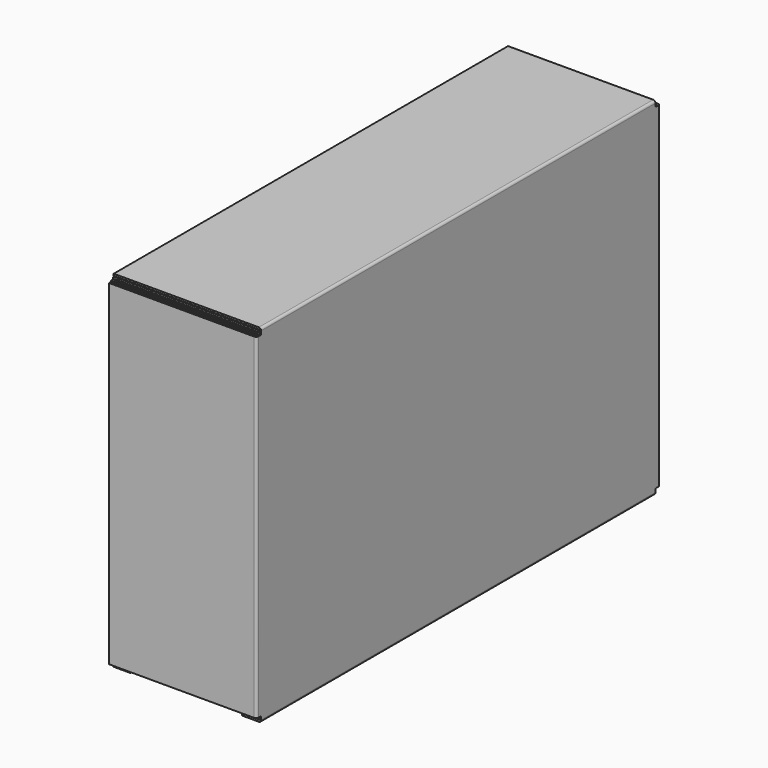
from build123d import *

# Parameters (mm, degrees)
F0_W      = 1092.2
F0_H      = 749.3
F1_DEPTH  = 317.5
F2_T      = -4.064
F3_W      = 279.4
F3_H      = 1717.7925925926
F4_DEPTH  = 4.064
F6_DEPTH  = 317.501
F7_R      = 2.54
F8_W      = 1084.072
F8_H      = 12.7
F9_DEPTH  = 313.436
F10_DEPTH = 317.5
F11_T     = 4.064
F13_DEPTH = 321.565
F14_R     = 5.08
F15_W     = 279.4
F15_H     = 1074.928
F16_DEPTH = 25.4


with BuildPart() as f1:
    # F0 (on Right) → F1 (new body)
    with BuildSketch(Plane.YZ):
        with Locations((546.1, 374.65)):
            Rectangle(F0_W, F0_H)
    extrude(amount=F1_DEPTH)

    # F2
    f2_openings = [f1.faces().sort_by_distance(p)[0] for p in [
        (317.5, 546.1, 374.65),
    ]]
    offset(amount=F2_T, openings=f2_openings)

    # F3 (on face) → F4 (cut)
    with BuildSketch(Plane(origin=(0, 0, 0), x_dir=(1, 0, 0), z_dir=(0, 0, -1))):
        with Locations((177.8, -858.8962962963)):
            Rectangle(F3_W, F3_H)
    extrude(amount=-F4_DEPTH, mode=Mode.SUBTRACT)

    # F5 (on face) → F6 (cut, through all)
    with BuildSketch(Plane(origin=(0, 0, 0), x_dir=(0, -1, 0), z_dir=(-1, 0, 0))):
        with BuildLine():
            Line((-1092.2, 6.35), (-1092.2, 0))
            Line((-1092.2, 0), (-1085.85, 0))
            Line((-1085.85, 0), (-1085.85, 3.81))
            ThreePointArc((-1085.85, 3.81), (-1086.5939487758, 5.6060512242), (-1088.39, 6.35))
            Line((-1088.39, 6.35), (-1092.2, 6.35))
        make_face()
        with BuildLine():
            Line((-1085.85, 749.3), (-1092.2, 749.3))
            Line((-1092.2, 749.3), (-1092.2, 742.95))
            Line((-1092.2, 742.95), (-1088.39, 742.95))
            ThreePointArc((-1088.39, 742.95), (-1086.5939487758, 743.6939487758), (-1085.85, 745.49))
            Line((-1085.85, 745.49), (-1085.85, 749.3))
        make_face()
        with BuildLine():
            Line((0, 742.95), (0, 749.3))
            Line((0, 749.3), (-6.35, 749.3))
            Line((-6.35, 749.3), (-6.35, 745.49))
            ThreePointArc((-6.35, 745.49), (-5.6060512242, 743.6939487758), (-3.81, 742.95))
            Line((-3.81, 742.95), (0, 742.95))
        make_face()
        with BuildLine():
            Line((-6.35, 0), (0, 0))
            Line((0, 0), (0, 6.35))
            Line((0, 6.35), (-3.81, 6.35))
            ThreePointArc((-3.81, 6.35), (-5.6060512242, 5.6060512242), (-6.35, 3.81))
            Line((-6.35, 3.81), (-6.35, 0))
        make_face()
    extrude(amount=-F6_DEPTH, mode=Mode.SUBTRACT)

    # F7
    f7_edges = [f1.edges().sort_by_distance(p)[0] for p in [
        (0, 1092.2, 374.65),
        (0, 546.1, 0),
        (0, 0, 374.65),
        (0, 546.1, 749.3),
    ]]
    fillet(f7_edges, radius=F7_R)


with BuildPart() as f9:
    # F8 (on face) → F9 (new body, through all)
    with BuildSketch(Plane.YZ.offset(4.064)):
        with Locations((546.1, 10.414)):
            Rectangle(F8_W, F8_H)
    extrude(amount=F9_DEPTH)


with BuildPart() as f10:
    # F0 (on Right) → F10 (new body)
    with BuildSketch(Plane.YZ):
        with Locations((546.1, 374.65)):
            Rectangle(F0_W, F0_H)
    extrude(amount=F10_DEPTH)

    # F11
    f11_openings = [f10.faces().sort_by_distance(p)[0] for p in [
        (0, 546.1, 374.65),
    ]]
    offset(amount=F11_T, openings=f11_openings, kind=Kind.INTERSECTION)

    # F12 (on face) → F13 (cut, through all)
    with BuildSketch(Plane.YZ.offset(321.564)):
        with BuildLine():
            Line((1083.564, -4.064), (1096.264, -4.064))
            Line((1096.264, -4.064), (1096.264, 8.636))
            Line((1096.264, 8.636), (1086.104, 8.636))
            ThreePointArc((1086.104, 8.636), (1084.3079487758, 7.8920512242), (1083.564, 6.096))
            Line((1083.564, 6.096), (1083.564, -4.064))
        make_face()
        with BuildLine():
            Line((8.636, 753.364), (-4.064, 753.364))
            Line((-4.064, 753.364), (-4.064, 740.664))
            Line((-4.064, 740.664), (6.096, 740.664))
            ThreePointArc((6.096, 740.664), (7.8920512242, 741.4079487758), (8.636, 743.204))
            Line((8.636, 743.204), (8.636, 753.364))
        make_face()
        with BuildLine():
            Line((1096.264, 740.664), (1096.264, 753.364))
            Line((1096.264, 753.364), (1083.564, 753.364))
            Line((1083.564, 753.364), (1083.564, 743.204))
            ThreePointArc((1083.564, 743.204), (1084.3079487758, 741.4079487758), (1086.104, 740.664))
            Line((1086.104, 740.664), (1096.264, 740.664))
        make_face()
        with BuildLine():
            Line((-4.064, 8.636), (-4.064, -4.064))
            Line((-4.064, -4.064), (8.636, -4.064))
            Line((8.636, -4.064), (8.636, 6.096))
            ThreePointArc((8.636, 6.096), (7.8920512242, 7.8920512242), (6.096, 8.636))
            Line((6.096, 8.636), (-4.064, 8.636))
        make_face()
    extrude(amount=-F13_DEPTH, mode=Mode.SUBTRACT)

    # F14
    f14_edges = [f10.edges().sort_by_distance(p)[0] for p in [
        (321.564, -4.064, 374.65),
        (321.564, 1096.264, 374.65),
        (321.564, 546.1, -4.064),
        (321.564, 546.1, 753.364),
    ]]
    fillet(f14_edges, radius=F14_R)

    # F15 (on face) → F16 (cut)
    with BuildSketch(Plane(origin=(0, 0, -4.064), x_dir=(1, 0, 0), z_dir=(0, 0, -1))):
        with Locations((139.7, -546.1)):
            Rectangle(F15_W, F15_H)
    extrude(amount=-F16_DEPTH, mode=Mode.SUBTRACT)


solid = Compound([f1.part, f9.part, f10.part])
